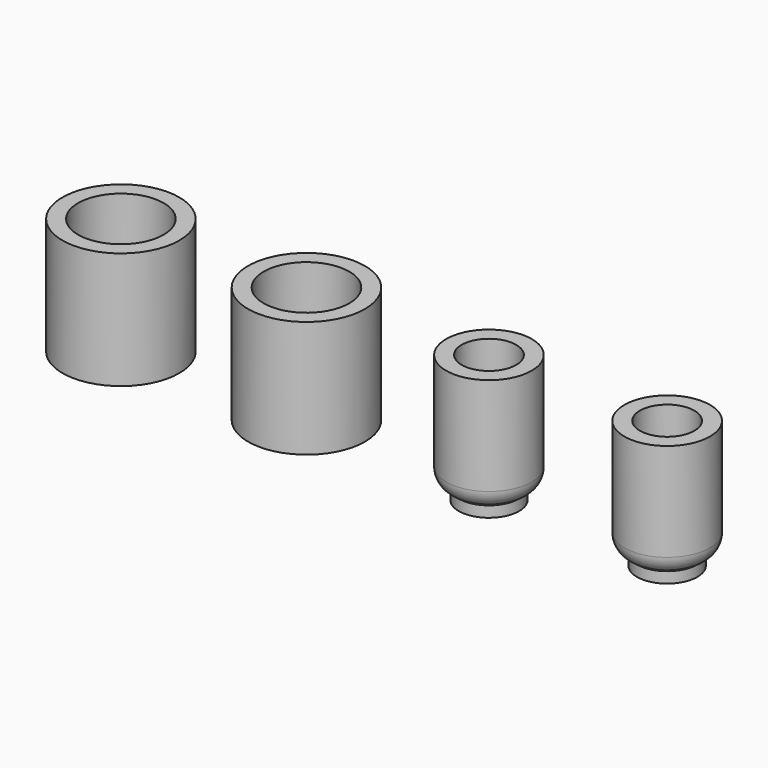
from build123d import *

# Parameters (mm, degrees)
F0_R      = 9.525
F1_DEPTH  = 19.05
F2_T      = -2.54
F3_R      = 7.4675144066
F4_DEPTH  = 1.778
F6_R      = 9.525
F7_DEPTH  = 19.05
F8_T      = -2.54
F9_R      = 7.4675111
F10_DEPTH = 1.778
F12_R     = 6.985
F13_DEPTH = 19.05
F14_T     = -2.54
F14_2_T   = -2.54
F15_R     = 4.9274984
F17_DEPTH = 1.778
F16_R     = 4.9274984
F18_R     = 3.0660512242
F19_R     = 3.0734


# Not quite as in the source:
# - a fillet or chamfer that OpenCascade refuses, or shapes differently, is made with other operations: its cross-section is extruded or revolved along the edge and cut away or added


with BuildPart() as f1:
    # F0 (on Top) → F1 (new body)
    with BuildSketch(Plane.XY):
        Circle(F0_R)
    extrude(amount=F1_DEPTH)

    # F2
    f2_openings = [f1.faces().sort_by_distance(p)[0] for p in [
        (0, 0, 19.05),
    ]]
    offset(amount=F2_T, openings=f2_openings)

    # F3 (on face) → F4 (join)
    with BuildSketch(Plane(origin=(0, 0, 0), x_dir=(1, 0, 0), z_dir=(0, 0, -1))):
        Circle(F3_R)
    extrude(amount=F4_DEPTH)

    # F5: fillet of radius 5.08 on 1 edges, made by hand

    # F5_s1 → F5_t2 (revolve, cut)
    with BuildSketch(Plane.XZ):
        with BuildLine():
            ThreePointArc((7.4675144066, 0), (5.732165099, -1.3121391396), (3.6070486316, -1.778))
            Line((3.6070486316, -1.778), (7.4675144066, -1.778))
            Line((7.4675144066, -1.778), (7.4675144066, 0))
        make_face()
    revolve(axis=Axis((0, 0, -1.778), (0, 0, -1)), mode=Mode.SUBTRACT)


with BuildPart() as f7:
    # F6 (on Top) → F7 (new body)
    with BuildSketch(Plane.XY):
        with Locations((-30.2620413402, 0)):
            Circle(F6_R)
    extrude(amount=F7_DEPTH)

    # F8
    f8_openings = [f7.faces().sort_by_distance(p)[0] for p in [
        (-30.262041, 0, 19.05),
    ]]
    offset(amount=F8_T, openings=f8_openings)

    # F9 (on face) → F10 (join)
    with BuildSketch(Plane(origin=(0, 0, 0), x_dir=(1, 0, 0), z_dir=(0, 0, -1))):
        with Locations((-30.2620413402, 0)):
            Circle(F9_R)
    extrude(amount=F10_DEPTH)

    # F11: fillet of radius 5.08 on 1 edges, made by hand

    # F11_s1 → F11_t2 (revolve, cut)
    with BuildSketch(Plane.XZ):
        with BuildLine():
            ThreePointArc((-22.7945302402, 0), (-24.5298795478, -1.3121391396), (-26.6549960152, -1.778))
            Line((-26.6549960152, -1.778), (-22.7945302402, -1.778))
            Line((-22.7945302402, -1.778), (-22.7945302402, 0))
        make_face()
    revolve(axis=Axis((-30.2620413402, 0, -1.778), (0, 0, -1)), mode=Mode.SUBTRACT)


with BuildPart() as f13:
    # F12 (on Top) → F13 (new body)
    with BuildSketch(Plane.XY):
        with Locations((29.7524470468, 0)):
            Circle(F12_R)
    extrude(amount=F13_DEPTH)

    # F14#2
    f14_2_openings = [f13.faces().sort_by_distance(p)[0] for p in [
        (29.752447, 0, 19.05),
    ]]
    offset(amount=F14_2_T, openings=f14_2_openings)

    # F19
    f19_edges = [f13.edges().sort_by_distance(p)[0] for p in [
        (22.767447, 0, 0),
    ]]
    fillet(f19_edges, radius=F19_R)


with BuildPart() as f13b:
    # F12 (on Top) → F13, piece 2 (new body)
    with BuildSketch(Plane.XY):
        with Locations((58.8081218302, 0)):
            Circle(F12_R)
    extrude(amount=F13_DEPTH)

    # F14
    f14_openings = [f13b.faces().sort_by_distance(p)[0] for p in [
        (58.808122, 0, 19.05),
    ]]
    offset(amount=F14_T, openings=f14_openings)

    # F18
    f18_edges = [f13b.edges().sort_by_distance(p)[0] for p in [
        (51.823122, 0, 0),
    ]]
    fillet(f18_edges, radius=F18_R)


with BuildPart() as f17:
    # F15 (on face) → F17 (new body)
    with BuildSketch(Plane(origin=(0, 0, 0), x_dir=(1, 0, 0), z_dir=(0, 0, -1))):
        with Locations((29.7524470468, 0)):
            Circle(F15_R)
    extrude(amount=F17_DEPTH)


with BuildPart() as f17b:
    # F16 (on face) → F17, piece 2 (new body)
    with BuildSketch(Plane(origin=(0, 0, 0), x_dir=(1, 0, 0), z_dir=(0, 0, -1))):
        with Locations((58.8081218302, 0)):
            Circle(F16_R)
    extrude(amount=F17_DEPTH)


solid = Compound([f1.part, f7.part, f13.part, f13b.part, f17.part, f17b.part])
